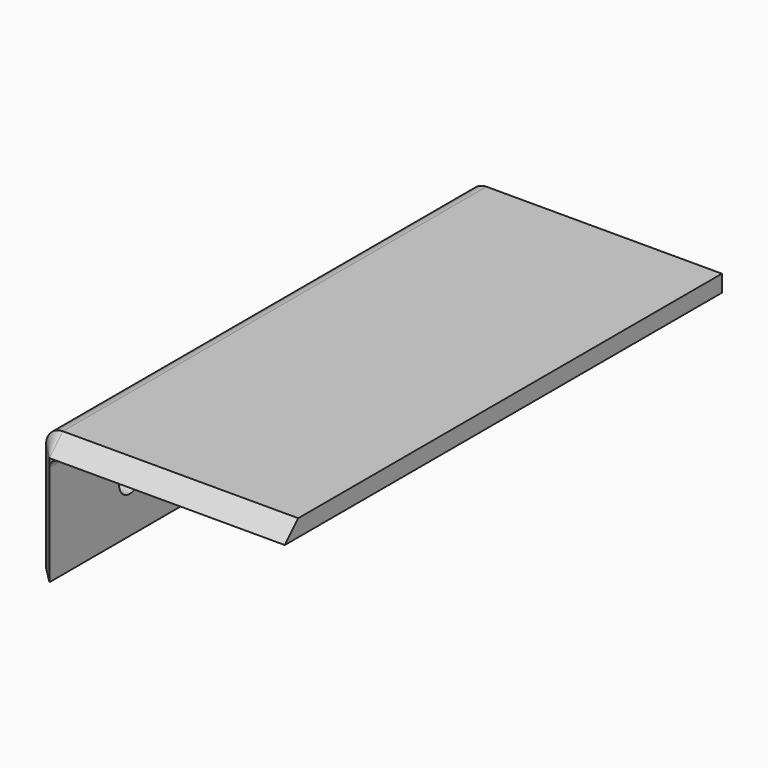
from build123d import *

# Parameters (mm, degrees)
F1_DEPTH = 65
F2_SIZE  = 1.99999
F3_R     = 1.6
F4_DEPTH = 2


# Not quite as in the source:
# - a fillet or chamfer is up to 0.001 mm smaller than in the source, because OpenCascade refuses the exact size


with BuildPart() as f1:
    # F0 (on Front) → F1 (new body)
    with BuildSketch(Plane.XZ):
        with BuildLine():
            Line((-16.8549300951, -0.3802398592), (-16.8549300951, -13.3802398592))
            Line((-16.8549300951, -13.3802398592), (-14.8549300951, -13.3802398592))
            Line((-14.8549300951, -13.3802398592), (-14.8549300951, -1.3802398592))
            ThreePointArc((-14.8549300951, -1.3802398592), (-14.5620368763, -0.673133078), (-13.8549300951, -0.3802398592))
            Line((-13.8549300951, -0.3802398592), (13.1450699049, -0.3802398592))
            Line((13.1450699049, -0.3802398592), (13.1450699049, 1.6197601408))
            Line((13.1450699049, 1.6197601408), (-14.8549300951, 1.6197601408))
            ThreePointArc((-14.8549300951, 1.6197601408), (-16.2691436574, 1.0339737031), (-16.8549300951, -0.3802398592))
        make_face()
    extrude(amount=F1_DEPTH)

    # F2 (size 2 in the source; OpenCascade refuses exactly that, so slightly less here)
    f2_edges = [f1.edges().sort_by_distance(p)[0] for p in [
        (-16.85493, -65, -6.88024),
    ]]
    chamfer(f2_edges, length=F2_SIZE)

    # F3 (on face) → F4 (cut, through all)
    with BuildSketch(Plane.YZ.offset(-14.8549300951)):
        with Locations((-53.0466809869, -7.3802398592)):
            Circle(F3_R)
        with Locations((-11.9533190131, -7.3802398592)):
            Circle(F3_R)
    extrude(amount=-F4_DEPTH, mode=Mode.SUBTRACT)


solid = f1.part
